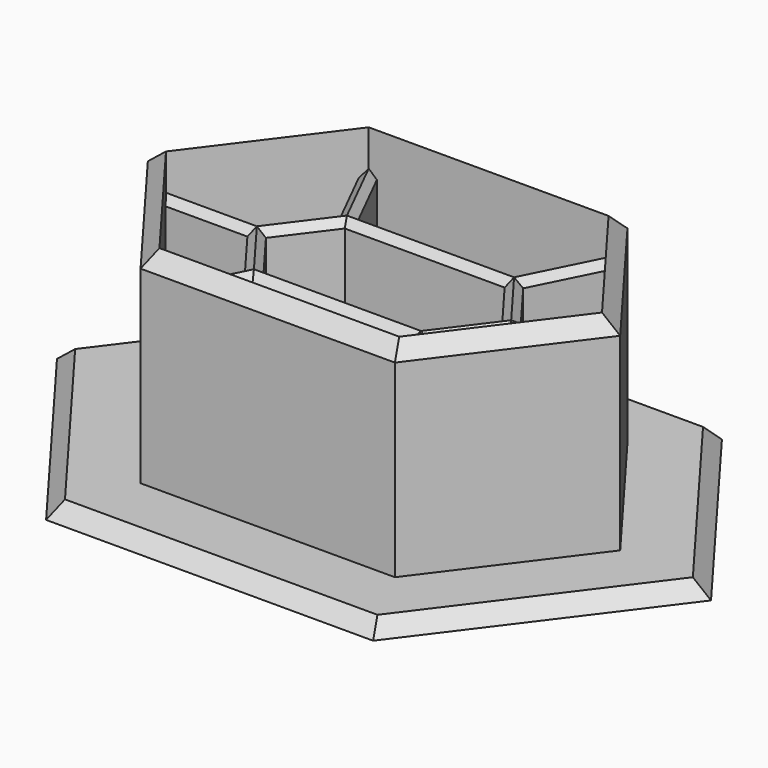
from build123d import *

# Parameters (mm, degrees)
F1_DEPTH = 30
F2_DEPTH = 2
F3_SIZE  = 1.99999
F5_DEPTH = 25
F6_SIZE  = 0.99999


# Not quite as in the source:
# - a fillet or chamfer is up to 0.001 mm smaller than in the source, because OpenCascade refuses the exact size


with BuildPart() as f1:
    # F0 (on Top) → F1 (new body)
    with BuildSketch(Plane.XY):
        Polygon((17.5, 20), (-17.5, 20), (-32.5, 0), (-17.5, -20), (17.5, -20), (32.5, 0), align=None)
        Polygon((16.5, -18), (-16.5, -18), (-30, 0), (-16.5, 18), (16.5, 18), (30, 0), align=None, mode=Mode.SUBTRACT)
    extrude(amount=F1_DEPTH)

    # F0 (on Top) → F2 (join)
    with BuildSketch(Plane.XY):
        Polygon((-45, 0), (-22.5, -30), (22.5, -30), (45, 0), (22.5, 30), (-22.5, 30), align=None)
        Polygon((-32.5, 0), (-17.5, 20), (17.5, 20), (32.5, 0), (17.5, -20), (-17.5, -20), align=None, mode=Mode.SUBTRACT)
    extrude(amount=F2_DEPTH)

    # F3 (size 2 in the source; OpenCascade refuses exactly that, so slightly less here)
    f3_edges = [f1.edges().sort_by_distance(p)[0] for p in [
        (-25, 10, 30),
        (0, 20, 30),
        (25, 10, 30),
        (25, -10, 30),
        (0, -20, 30),
        (-25, -10, 30),
        (0, -30, 2),
        (33.75, -15, 2),
        (33.75, 15, 2),
        (-33.75, -15, 2),
        (-33.75, 15, 2),
        (0, 30, 2),
    ]]
    chamfer(f3_edges, length=F3_SIZE)

    # F4 (on Top) → F5 (join)
    with BuildSketch(Plane.XY):
        Polygon((-17.1708203932, -17.105572809), (-16.5, -18), (-15.3819660113, -18), (-10.8819660113, -9), (10.8819660113, -9), (15.3819660113, -18), (16.5, -18), (17.1708203932, -17.105572809), (12.6708203932, -8.105572809), (18, -1), (29.25, -1), (30, 0), (29.25, 1), (18, 1), (12.6708203932, 8.105572809), (17.1708203932, 17.105572809), (16.5, 18), (15.3819660113, 18), (10.8819660113, 9), (-10.8819660113, 9), (-15.3819660113, 18), (-16.5, 18), (-17.1708203932, 17.105572809), (-12.6708203932, 8.105572809), (-18, 1), (-29.25, 1), (-30, 0), (-29.25, -1), (-18, -1), (-12.6708203932, -8.105572809), align=None)
        Polygon((-11, -7), (-16.25, 0), (-11, 7), (11, 7), (16.25, 0), (11, -7), align=None, mode=Mode.SUBTRACT)
    extrude(amount=F5_DEPTH)

    # F6 (size 1 in the source; OpenCascade refuses exactly that, so slightly less here)
    f6_edges = [f1.edges().sort_by_distance(p)[0] for p in [
        (-23.625, -1, 25),
        (-23.625, 1, 25),
        (-15.33541, -4.552786, 25),
        (-13.625, -3.5, 25),
        (-13.625, 3.5, 25),
        (-15.33541, 4.552786, 25),
        (-14.92082, 12.605573, 25),
        (-13.131966, 13.5, 25),
        (0, 7, 25),
        (0, 9, 25),
        (0, -9, 25),
        (0, -7, 25),
        (-13.131966, -13.5, 25),
        (-14.92082, -12.605573, 25),
        (14.92082, -12.605573, 25),
        (13.131966, -13.5, 25),
        (15.33541, -4.552786, 25),
        (13.625, -3.5, 25),
        (23.625, -1, 25),
        (23.625, 1, 25),
        (15.33541, 4.552786, 25),
        (13.625, 3.5, 25),
        (14.92082, 12.605573, 25),
        (13.131966, 13.5, 25),
    ]]
    chamfer(f6_edges, length=F6_SIZE)


solid = f1.part
